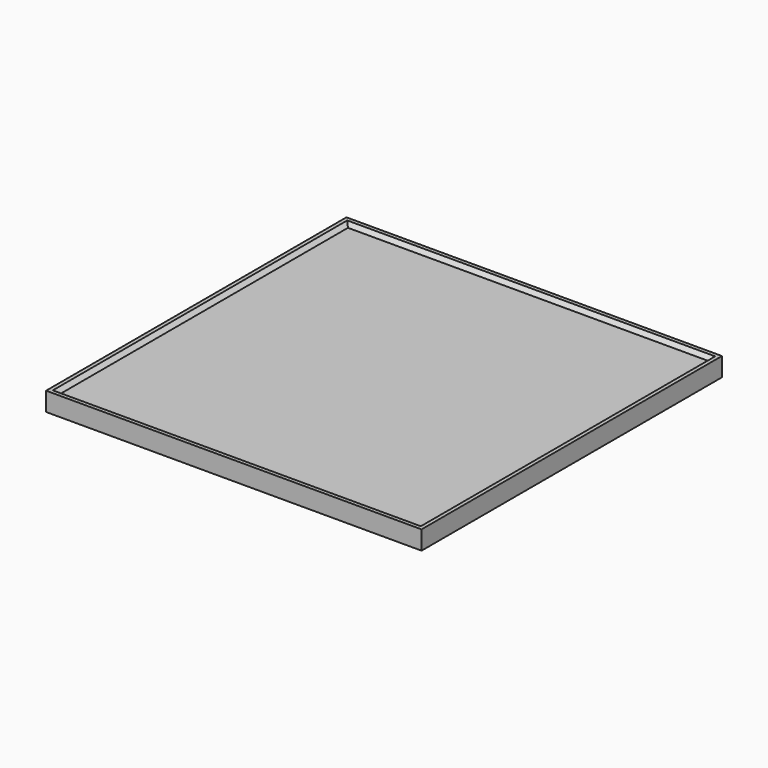
from build123d import *

# Parameters (mm, degrees)
F0_W     = 500
F0_H     = 500
F1_DEPTH = 25
F2_W     = 490.0000095367
F2_H     = 490.0000095367
F3_DEPTH = 5
F4_SIZE  = 4.99999


# Not quite as in the source:
# - a fillet or chamfer is up to 0.001 mm smaller than in the source, because OpenCascade refuses the exact size


with BuildPart() as f1:
    # F0 (on Top) → F1 (new body)
    with BuildSketch(Plane.XY):
        Rectangle(F0_W, F0_H)
    extrude(amount=F1_DEPTH)

    # F2 (on face) → F3 (cut)
    with BuildSketch(Plane.XY.offset(25)):
        Rectangle(F2_W, F2_H)
    extrude(amount=-F3_DEPTH, mode=Mode.SUBTRACT)

    # F4 (size 5 in the source; OpenCascade refuses exactly that, so slightly less here)
    f4_edges = [f1.edges().sort_by_distance(p)[0] for p in [
        (0, -245.000005, 20),
        (245.000005, 0, 20),
        (0, 245.000005, 20),
        (-245.000005, 0, 20),
    ]]
    chamfer(f4_edges, length=F4_SIZE)


solid = f1.part
